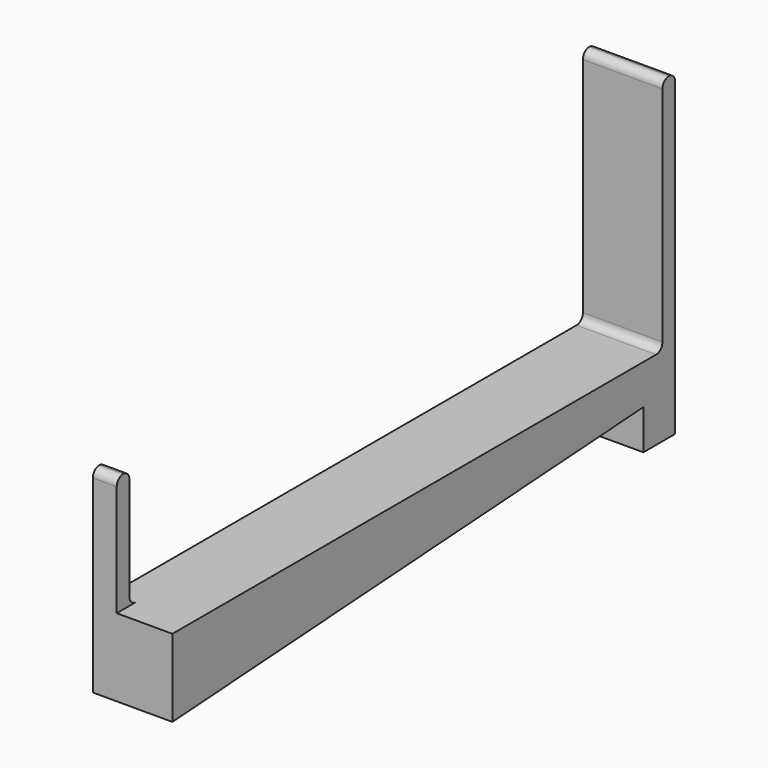
from build123d import *

# Parameters (mm, degrees)
F0_W      = 10
F0_H      = 79
F1_DEPTH  = 10
F2_W      = 10
F2_H      = 2
F3_DEPTH  = 15
F4_W      = 10
F4_H      = 2
F5_DEPTH  = 30
F7_DEPTH  = 10.001
F8_R      = 0.99999
F9_W      = 4.9229283333
F9_H      = 15
F10_DEPTH = 7


# Not quite as in the source:
# - a fillet or chamfer is up to 0.001 mm smaller than in the source, because OpenCascade refuses the exact size


with BuildPart() as f1:
    # F0 (on Top) → F1 (new body)
    with BuildSketch(Plane.XY):
        Rectangle(F0_W, F0_H)
    extrude(amount=F1_DEPTH)

    # F2 (on face) → F3 (join)
    with BuildSketch(Plane.XY.offset(10)):
        with Locations((0, -38.5)):
            Rectangle(F2_W, F2_H)
    extrude(amount=F3_DEPTH)

    # F4 (on face) → F5 (join)
    with BuildSketch(Plane.XY.offset(10)):
        with Locations((0, 38.5)):
            Rectangle(F4_W, F4_H)
    extrude(amount=F5_DEPTH)

    # F6 (on face) → F7 (cut, through all)
    with BuildSketch(Plane.YZ.offset(5)):
        Polygon((34.5, 5), (-43.3395786217, 0), (34.5, 0), align=None)
    extrude(amount=-F7_DEPTH, mode=Mode.SUBTRACT)

    # F8 (radius 1 in the source; OpenCascade refuses exactly that, so slightly less here)
    f8_edges = [f1.edges().sort_by_distance(p)[0] for p in [
        (0, -39.5, 25),
        (0, -37.5, 25),
        (0, 37.5, 40),
        (0, 39.5, 40),
        (0, -37.5, 10),
        (0, 37.5, 10),
    ]]
    fillet(f8_edges, radius=F8_R)

    # F9 (on face) → F10 (cut)
    with BuildSketch(Plane.YZ.offset(5)):
        with Locations((-37.0385358334, 17.5)):
            Rectangle(F9_W, F9_H)
    extrude(amount=-F10_DEPTH, mode=Mode.SUBTRACT)


solid = f1.part
